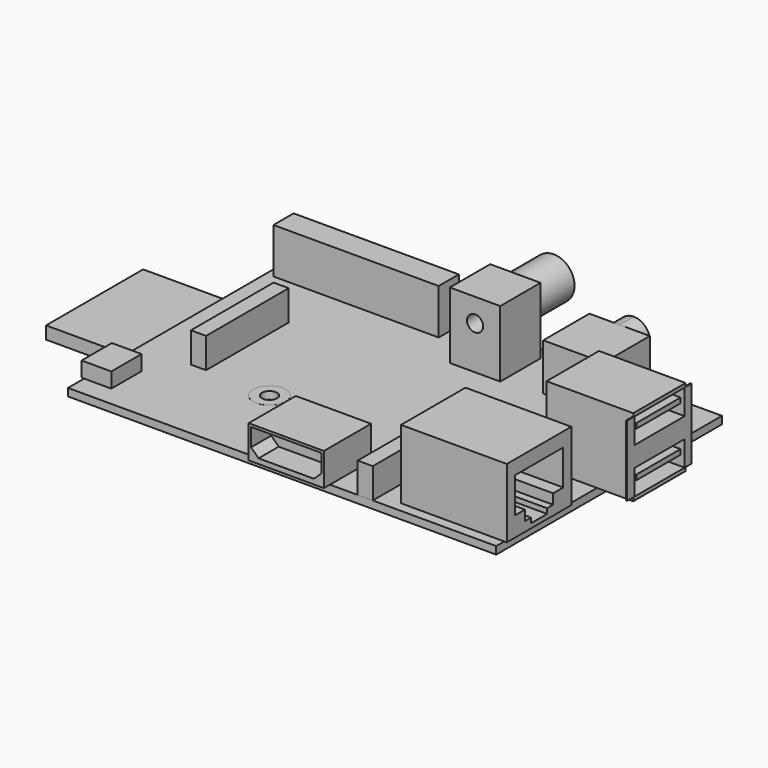
from build123d import *

# Parameters (mm, degrees)
F0_R      = 3.25
F0_W      = 32.8
F0_H      = 5
F0_W_2    = 10
F0_H_2    = 10
F0_H_3    = 13
F0_R_2    = 1.5
F0_W_3    = 20.5
F0_H_4    = 16
F0_W_4    = 13.5
F0_H_5    = 24
F0_W_5    = 3.0046645552
F0_H_6    = 20.5
F0_W_6    = 1
F0_W_7    = 5.4
F0_H_7    = 7.5
F0_W_8    = 12
F0_H_8    = 11.4661744535
F0_W_9    = 14.9416802451
F0_H_9    = 10.2
F0_W_10   = 3
F0_H_10   = 22
F1_DEPTH  = 1.5
F0_W_11   = 0.5
F2_DEPTH  = 13.7
F0_W_12   = 7
F3_DEPTH  = 15.4
F4_DEPTH  = 9.3
F5_DEPTH  = 13.2
F6_DEPTH  = 9
F7_DEPTH  = 6
F0_H_11   = 1.5
F8_DEPTH  = 6.5
F9_DEPTH  = 0.01
F10_DEPTH = 3
F11_DEPTH = 6
F13_DEPTH = 3.7
F12_W     = 13.7211494148
F12_H     = 24.080616422
F12_W_2   = 0.8938605189
F12_W_3   = 17.5610897839
F14_DEPTH = 2.5
F15_R     = 1.75
F16_DEPTH = 3.5
F17_DEPTH = 10
F18_R     = 1.6
F19_DEPTH = 55.001
F18_R_2   = 3.15
F20_DEPTH = 9.5
F18_R_3   = 4.15
F21_DEPTH = 9.5
F23_DEPTH = 5
F25_DEPTH = 11
F27_DEPTH = 7
F29_DEPTH = 3
F30_W     = 1.5
F30_H     = 14
F26_W     = 13
F26_H     = 15.4
F31_DEPTH = 0.2


with BuildPart() as f1:
    # F0 (on Top) → F1 (new body)
    with BuildSketch(Plane.XY):
        Polygon((10.999614042, 28), (-47.700385958, 28), (-47.700385958, 12.6100301519), (-46.700385958, 12.6100301519), (-46.700385958, 14.1100301519), (-29.700385958, 14.1100301519), (-29.700385958, -13.8899698481), (-46.700385958, -13.8899698481), (-46.700385958, -11.3899698481), (-47.700385958, -11.3899698481), (-47.700385958, -16.5), (-42.300385958, -16.5), (-42.300385958, -24), (-47.700385958, -24), (-47.700385958, -28), (-10.6420662031, -28), (-10.6420662031, -17.8), (4.299614042, -17.8), (4.299614042, -28), (9.799614042, -28), (9.799614042, -6), (12.799614042, -6), (12.799614042, -28), (37.299614042, -28), (37.299614042, -26), (16.799614042, -26), (16.799614042, -10), (37.299614042, -10), (37.299614042, -3), (27.299614042, -3), (27.299614042, 10), (37.299614042, 10), (37.299614042, 28), (22.999614042, 28), (22.999614042, 16.5338255465), (10.999614042, 16.5338255465), align=None)
        with Locations((-21.700385958, -10.5)):
            Circle(F0_R, mode=Mode.SUBTRACT)
        with Locations((-29.800385958, 23.6)):
            Rectangle(F0_W, F0_H, mode=Mode.SUBTRACT)
        with Locations((-1.700385958, 20.5)):
            Rectangle(F0_W_2, F0_H_2, mode=Mode.SUBTRACT)
        with Locations((32.299614042, 15.5)):
            Circle(F0_R, mode=Mode.SUBTRACT)
        with Locations((32.299614042, 3.5)):
            Rectangle(F0_W_2, F0_H_3)
        with Locations((32.299614042, 15.5)):
            Circle(F0_R)
        with Locations((32.299614042, 15.5)):
            Circle(F0_R_2, mode=Mode.SUBTRACT)
        with Locations((-21.700385958, -10.5)):
            Circle(F0_R)
        with Locations((-21.700385958, -10.5)):
            Circle(F0_R_2, mode=Mode.SUBTRACT)
        with Locations((27.049614042, -18)):
            Rectangle(F0_W_3, F0_H_4)
        Polygon((-46.700385958, 14.1100301519), (-46.700385958, 12.6100301519), (-33.200385958, 12.6100301519), (-33.200385958, -11.3899698481), (-46.700385958, -11.3899698481), (-46.700385958, -13.8899698481), (-29.700385958, -13.8899698481), (-29.700385958, 14.1100301519), align=None)
        with Locations((-39.950385958, 0.6100301519)):
            Rectangle(F0_W_4, F0_H_5)
        with Locations((-36.1980536804, 0.25)):
            Rectangle(F0_W_5, F0_H_6, mode=Mode.SUBTRACT)
        with Locations((-47.200385958, 0.6100301519)):
            Rectangle(F0_W_6, F0_H_5)
        with Locations((-45.000385958, -20.25)):
            Rectangle(F0_W_7, F0_H_7)
        with Locations((-29.800385958, 23.6)):
            Rectangle(F0_W, F0_H)
        with Locations((-1.700385958, 20.5)):
            Rectangle(F0_W_2, F0_H_2)
        with Locations((16.999614042, 22.2669127733)):
            Rectangle(F0_W_8, F0_H_8)
        with Locations((-3.1712260805, -22.9)):
            Rectangle(F0_W_9, F0_H_9)
        with Locations((11.299614042, -17)):
            Rectangle(F0_W_10, F0_H_10)
        with Locations((-36.1980536804, 0.25)):
            Rectangle(F0_W_5, F0_H_6)
    extrude(amount=-F1_DEPTH)


with BuildPart() as f2:
    # F0 (on Top) → F2 (new body)
    with BuildSketch(Plane.XY):
        with Locations((27.049614042, -18)):
            Rectangle(F0_W_3, F0_H_4)
        with Locations((37.549614042, -18)):
            Rectangle(F0_W_11, F0_H_4)
    extrude(amount=F2_DEPTH)

    # F24 (on face) → F25 (cut)
    with BuildSketch(Plane.YZ.offset(37.799614042)):
        Polygon((-12, 10.9), (-18, 10.9), (-24, 10.9), (-24, 3.9), (-21.5, 3.9), (-21.5, 1.9), (-20, 1.9), (-20, 0.9), (-18, 0.9), (-16, 0.9), (-16, 1.9), (-14.5, 1.9), (-14.5, 3.9), (-12, 3.9), align=None)
    extrude(amount=-F25_DEPTH, mode=Mode.SUBTRACT)


with BuildPart() as f3:
    # F0 (on Top) → F3 (new body)
    with BuildSketch(Plane.XY):
        with Locations((32.299614042, 3.5)):
            Rectangle(F0_W_2, F0_H_3)
        with Locations((40.799614042, 3.5)):
            Rectangle(F0_W_12, F0_H_3)
    extrude(amount=F3_DEPTH)

    # F26 (on face) → F27 (cut)
    with BuildSketch(Plane.YZ.offset(44.299614042)):
        Polygon((9.75, 14.7), (3.5, 14.7), (-2.75, 14.7), (-2.75, 9.7), (3.5, 9.7), (9.75, 9.7), align=None)
        Polygon((-2, 13.2), (3.5, 13.2), (9, 13.2), (9, 12.2), (3.5, 12.2), (-2, 12.2), align=None, mode=Mode.SUBTRACT)
        Polygon((9.75, 5.7), (3.5, 5.7), (-2.75, 5.7), (-2.75, 0.7), (3.5, 0.7), (9.75, 0.7), align=None)
        Polygon((-2, 4.2), (3.5, 4.2), (9, 4.2), (9, 3.2), (3.5, 3.2), (-2, 3.2), align=None, mode=Mode.SUBTRACT)
    extrude(amount=-F27_DEPTH, mode=Mode.SUBTRACT)

    # F30 (on face) + F26 (on face) → F31 (join)
    with BuildSketch(Plane.YZ.offset(44.299614042)):
        with Locations((-3.75, 7.7)):
            Rectangle(F30_W, F30_H)
        with Locations((10.75, 7.7)):
            Rectangle(F30_W, F30_H)
    with BuildSketch(Plane.YZ.offset(44.299614042)):
        with Locations((3.5, 7.7)):
            Rectangle(F26_W, F26_H)
        Polygon((-2.75, 5.7), (3.5, 5.7), (9.75, 5.7), (9.75, 0.7), (3.5, 0.7), (-2.75, 0.7), align=None, mode=Mode.SUBTRACT)
        Polygon((-2.75, 14.7), (3.5, 14.7), (9.75, 14.7), (9.75, 9.7), (3.5, 9.7), (-2.75, 9.7), align=None, mode=Mode.SUBTRACT)
    extrude(amount=F31_DEPTH)


with BuildPart() as f4:
    # F0 (on Top) → F4 (new body)
    with BuildSketch(Plane.XY):
        with Locations((16.999614042, 22.2669127733)):
            Rectangle(F0_W_8, F0_H_8)
    extrude(amount=F4_DEPTH)

    # F15 (on face) → F16 (join)
    with BuildSketch(Plane(origin=(0, 28, 0), x_dir=(-1, 0, 0), z_dir=(0, 1, 0))):
        with BuildLine():
            ThreePointArc((-16.999614042, 9.3), (-19.2977110809, 3.7519029611), (-13.749614042, 6.05))
            ThreePointArc((-13.749614042, 6.05), (-14.7015170032, 8.3480970389), (-16.999614042, 9.3))
        make_face()
        with Locations((-16.999614042, 6.05)):
            Circle(F15_R, mode=Mode.SUBTRACT)
    extrude(amount=F16_DEPTH)

    # F15 (on face) → F17 (cut)
    with BuildSketch(Plane(origin=(0, 28, 0), x_dir=(-1, 0, 0), z_dir=(0, 1, 0))):
        with Locations((-16.999614042, 6.05)):
            Circle(F15_R)
    extrude(amount=-F17_DEPTH, mode=Mode.SUBTRACT)


with BuildPart() as f5:
    # F0 (on Top) → F5 (new body)
    with BuildSketch(Plane.XY):
        with Locations((-1.700385958, 20.5)):
            Rectangle(F0_W_2, F0_H_2)
    extrude(amount=F5_DEPTH)

    # F18 (on face) → F19 (cut, through all)
    with BuildSketch(Plane(origin=(0, 25.5, 0), x_dir=(-1, 0, 0), z_dir=(0, 1, 0))):
        with Locations((1.700385958, 8.55)):
            Circle(F18_R)
    extrude(amount=-F19_DEPTH, mode=Mode.SUBTRACT)

    # F18 (on face) → F20 (join)
    with BuildSketch(Plane(origin=(0, 25.5, 0), x_dir=(-1, 0, 0), z_dir=(0, 1, 0))):
        with Locations((1.700385958, 8.55)):
            Circle(F18_R_2)
        with Locations((1.700385958, 8.55)):
            Circle(F18_R, mode=Mode.SUBTRACT)
    extrude(amount=F20_DEPTH)


with BuildPart() as f6:
    # F0 (on Top) → F6 (new body)
    with BuildSketch(Plane.XY):
        with Locations((-29.800385958, 23.6)):
            Rectangle(F0_W, F0_H)
    extrude(amount=F6_DEPTH)


with BuildPart() as f7:
    # F0 (on Top) → F7 (new body)
    with BuildSketch(Plane.XY):
        with Locations((11.299614042, -17)):
            Rectangle(F0_W_10, F0_H_10)
    extrude(amount=F7_DEPTH)


with BuildPart() as f8:
    # F0 (on Top) → F8 (new body)
    with BuildSketch(Plane.XY):
        with Locations((-3.1712260805, -22.9)):
            Rectangle(F0_W_9, F0_H_9)
        with Locations((-3.1712260805, -28.75)):
            Rectangle(F0_W_9, F0_H_11)
    extrude(amount=F8_DEPTH)

    # F22 (on face) → F23 (cut)
    with BuildSketch(Plane.XZ.offset(29.5)):
        Polygon((3.8287739195, 2.4324118094), (3.8287739195, 6), (-3.1712260805, 6), (-10.1712260805, 6), (-10.1712260805, 2.4324118094), (-8.6712260805, 1), (-3.1712260805, 1), (2.3287739195, 1), align=None)
    extrude(amount=-F23_DEPTH, mode=Mode.SUBTRACT)


with BuildPart() as f9:
    # F0 (on Top) → F9 (new body)
    with BuildSketch(Plane.XY):
        with Locations((32.299614042, 15.5)):
            Circle(F0_R)
        with Locations((32.299614042, 15.5)):
            Circle(F0_R_2, mode=Mode.SUBTRACT)
    extrude(amount=F9_DEPTH)


with BuildPart() as f9b:
    # F0 (on Top) → F9, piece 2 (new body)
    with BuildSketch(Plane.XY):
        with Locations((-21.700385958, -10.5)):
            Circle(F0_R)
        with Locations((-21.700385958, -10.5)):
            Circle(F0_R_2, mode=Mode.SUBTRACT)
    extrude(amount=F9_DEPTH)


with BuildPart() as f10:
    # F0 (on Top) → F10 (new body)
    with BuildSketch(Plane.XY):
        with Locations((-45.000385958, -20.25)):
            Rectangle(F0_W_7, F0_H_7)
        with Locations((-47.950385958, -20.25)):
            Rectangle(F0_W_11, F0_H_7)
    extrude(amount=F10_DEPTH)

    # F28 (on face) → F29 (cut)
    with BuildSketch(Plane(origin=(-48.200385958, 0, 0), x_dir=(0, -1, 0), z_dir=(-1, 0, 0))):
        Polygon((23.7, 2.7), (20.25, 2.7), (16.8, 2.7), (16.8, 1.6567406064), (17.75, 0.3), (20.25, 0.3), (22.75, 0.3), (23.7, 1.6567406064), align=None)
        Polygon((18.2, 2.1), (20.25, 2.1), (22.3, 2.1), (22.3, 1.8), (20.25, 1.8), (18.2, 1.8), align=None, mode=Mode.SUBTRACT)
    extrude(amount=-F29_DEPTH, mode=Mode.SUBTRACT)


with BuildPart() as f11:
    # F0 (on Top) → F11 (new body)
    with BuildSketch(Plane.XY):
        with Locations((-36.1980536804, 0.25)):
            Rectangle(F0_W_5, F0_H_6)
    extrude(amount=F11_DEPTH)


with BuildPart() as f13:
    # F12 (on face) → F13 (new body)
    with BuildSketch(Plane(origin=(0, 0, -1.5), x_dir=(1, 0, 0), z_dir=(0, 0, -1))):
        Polygon((-46.806525439, 13.9555186033), (-46.806525439, 11.4857107401), (-33.0853760242, 11.4857107401), (-33.0853760242, -12.5949056819), (-46.806525439, -12.5949056819), (-46.806525439, -14.1728390008), (-29.4492729008, -14.1728390008), (-29.4492729008, 13.9555186033), align=None)
    extrude(amount=F13_DEPTH)

    # F12 (on face) → F14 (join)
    with BuildSketch(Plane(origin=(0, 0, -1.5), x_dir=(1, 0, 0), z_dir=(0, 0, -1))):
        with Locations((-39.9459507316, -0.5545974709)):
            Rectangle(F12_W, F12_H)
        with Locations((-47.2534556985, -0.5545974709)):
            Rectangle(F12_W_2, F12_H)
        with Locations((-56.4809308499, -0.5545974709)):
            Rectangle(F12_W_3, F12_H)
    extrude(amount=F14_DEPTH)


with BuildPart() as f21:
    # F18 (on face) → F21 (new body)
    with BuildSketch(Plane(origin=(0, 25.5, 0), x_dir=(-1, 0, 0), z_dir=(0, 1, 0))):
        with Locations((1.700385958, 8.55)):
            Circle(F18_R_3)
        with Locations((1.700385958, 8.55)):
            Circle(F18_R_2, mode=Mode.SUBTRACT)
    extrude(amount=F21_DEPTH)


solid = Compound([f1.part, f2.part, f3.part, f4.part, f5.part, f6.part, f7.part, f8.part, f9.part, f9b.part, f10.part, f11.part, f13.part, f21.part])
